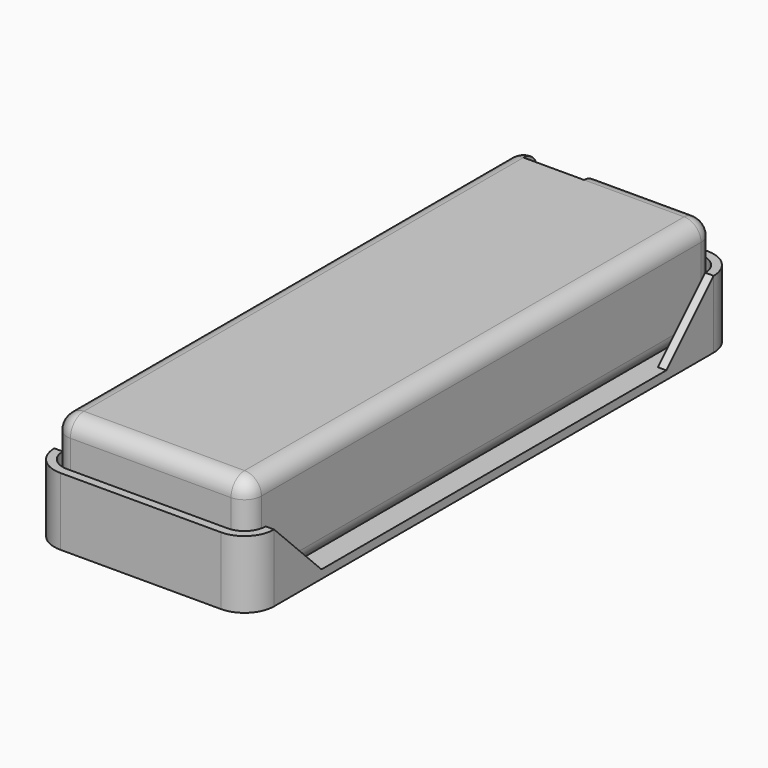
from build123d import *

# Parameters (mm, degrees)
F1_DEPTH  = 24
F2_R      = 4
F3_W      = 14.3697379231
F3_H      = 4.1815820932
F4_DEPTH  = 10
F5_DEPTH  = 14
F6_DEPTH  = 2
F7_DEPTH  = 2
F8_W      = 2
F8_H      = 130
F9_DEPTH  = 14
F10_DEPTH = 14
F11_DEPTH = 14
F12_SIZE  = 13.99999


# Not quite as in the source:
# - a fillet or chamfer is up to 0.001 mm smaller than in the source, because OpenCascade refuses the exact size


with BuildPart() as f1:
    # F0 (on Top) → F1 (new body)
    with BuildSketch(Plane.XY):
        with BuildLine():
            Line((-42, 0), (-4, 0))
            ThreePointArc((-4, 0), (-1.1715728753, 1.1715728753), (0, 4))
            Line((0, 4), (0, 134))
            ThreePointArc((0, 134), (-1.1715728753, 136.8284271247), (-4, 138))
            Line((-4, 138), (-42, 138))
            ThreePointArc((-42, 138), (-44.8284271247, 136.8284271247), (-46, 134))
            Line((-46, 134), (-46, 4))
            ThreePointArc((-46, 4), (-44.8284271247, 1.1715728753), (-42, 0))
        make_face()
    extrude(amount=F1_DEPTH)

    # F2
    f2_edges = [f1.edges().sort_by_distance(p)[0] for p in [
        (-46, 69, 24),
        (-44.828427, 1.171573, 24),
        (-23, 0, 24),
        (-1.171573, 1.171573, 24),
        (0, 69, 24),
        (-1.171573, 136.828427, 24),
        (-23, 138, 24),
        (-44.828427, 136.828427, 24),
        (-46, 69, 0),
        (-44.828427, 1.171573, 0),
        (-23, 0, 0),
        (-1.171573, 1.171573, 0),
        (0, 69, 0),
        (-1.171573, 136.828427, 0),
        (-23, 138, 0),
        (-44.828427, 136.828427, 0),
    ]]
    fillet(f2_edges, radius=F2_R)

    # F3 (on face) → F4 (cut)
    with BuildSketch(Plane.XY.offset(24)):
        with Locations((-34.8151310384, 136.0907910466)):
            Rectangle(F3_W, F3_H)
    extrude(amount=-F4_DEPTH, mode=Mode.SUBTRACT)


with BuildPart() as f5:
    # F0 (on Top) → F5 (new body)
    with BuildSketch(Plane.XY):
        with BuildLine():
            Line((-42, -3), (-4, -3))
            ThreePointArc((-4, -3), (0.9497474683, -0.9497474683), (3, 4))
            Line((3, 4), (3, 134))
            ThreePointArc((3, 134), (0.9497474683, 138.9497474683), (-4, 141))
            Line((-4, 141), (-42, 141))
            ThreePointArc((-42, 141), (-46.9497474683, 138.9497474683), (-49, 134))
            Line((-49, 134), (-49, 4))
            ThreePointArc((-49, 4), (-46.9497474683, -0.9497474683), (-42, -3))
        make_face()
        with BuildLine():
            ThreePointArc((-42, -1), (-45.5355339059, 0.4644660941), (-47, 4))
            Line((-47, 4), (-47, 134))
            ThreePointArc((-47, 134), (-45.5355339059, 137.5355339059), (-42, 139))
            Line((-42, 139), (-4, 139))
            ThreePointArc((-4, 139), (-0.4644660941, 137.5355339059), (1, 134))
            Line((1, 134), (1, 4))
            ThreePointArc((1, 4), (-0.4644660941, 0.4644660941), (-4, -1))
            Line((-4, -1), (-42, -1))
        make_face(mode=Mode.SUBTRACT)
    extrude(amount=F5_DEPTH)



with BuildPart() as f6:
    # F0 (on Top) → F6 (new body)
    with BuildSketch(Plane.XY):
        with BuildLine():
            Line((-42, -3), (-4, -3))
            ThreePointArc((-4, -3), (0.9497474683, -0.9497474683), (3, 4))
            Line((3, 4), (3, 134))
            ThreePointArc((3, 134), (0.9497474683, 138.9497474683), (-4, 141))
            Line((-4, 141), (-42, 141))
            ThreePointArc((-42, 141), (-46.9497474683, 138.9497474683), (-49, 134))
            Line((-49, 134), (-49, 4))
            ThreePointArc((-49, 4), (-46.9497474683, -0.9497474683), (-42, -3))
        make_face()
        with BuildLine():
            ThreePointArc((-42, -1), (-45.5355339059, 0.4644660941), (-47, 4))
            Line((-47, 4), (-47, 134))
            ThreePointArc((-47, 134), (-45.5355339059, 137.5355339059), (-42, 139))
            Line((-42, 139), (-4, 139))
            ThreePointArc((-4, 139), (-0.4644660941, 137.5355339059), (1, 134))
            Line((1, 134), (1, 4))
            ThreePointArc((1, 4), (-0.4644660941, 0.4644660941), (-4, -1))
            Line((-4, -1), (-42, -1))
        make_face(mode=Mode.SUBTRACT)
    extrude(amount=-F6_DEPTH)


with BuildPart() as f6b:
    # F0 (on Top) → F6, piece 2 (new body)
    with BuildSketch(Plane.XY):
        with BuildLine():
            Line((-42, 0), (-4, 0))
            ThreePointArc((-4, 0), (-1.1715728753, 1.1715728753), (0, 4))
            Line((0, 4), (0, 134))
            ThreePointArc((0, 134), (-1.1715728753, 136.8284271247), (-4, 138))
            Line((-4, 138), (-42, 138))
            ThreePointArc((-42, 138), (-44.8284271247, 136.8284271247), (-46, 134))
            Line((-46, 134), (-46, 4))
            ThreePointArc((-46, 4), (-44.8284271247, 1.1715728753), (-42, 0))
        make_face()
    extrude(amount=-F6_DEPTH)


with BuildPart() as f5_1:
    add(f5.part)

    add(f6.part)  # F7 merges F6

    add(f6b.part)  # F7 merges F6b
    # F0 (on Top) → F7 (join)
    with BuildSketch(Plane.XY):
        with BuildLine():
            Line((-47, 134), (-47, 4))
            ThreePointArc((-47, 4), (-45.5355339059, 0.4644660941), (-42, -1))
            Line((-42, -1), (-4, -1))
            ThreePointArc((-4, -1), (-0.4644660941, 0.4644660941), (1, 4))
            Line((1, 4), (1, 134))
            ThreePointArc((1, 134), (-0.4644660941, 137.5355339059), (-4, 139))
            Line((-4, 139), (-42, 139))
            ThreePointArc((-42, 139), (-45.5355339059, 137.5355339059), (-47, 134))
        make_face()
        with BuildLine():
            ThreePointArc((0, 4), (-1.1715728753, 1.1715728753), (-4, 0))
            Line((-4, 0), (-42, 0))
            ThreePointArc((-42, 0), (-44.8284271247, 1.1715728753), (-46, 4))
            Line((-46, 4), (-46, 134))
            ThreePointArc((-46, 134), (-44.8284271247, 136.8284271247), (-42, 138))
            Line((-42, 138), (-4, 138))
            ThreePointArc((-4, 138), (-1.1715728753, 136.8284271247), (0, 134))
            Line((0, 134), (0, 4))
        make_face(mode=Mode.SUBTRACT)
    extrude(amount=-F7_DEPTH)

    # F8 (on face) → F9 (cut)
    with BuildSketch(Plane.XY.offset(14)):
        with Locations((-48, 69)):
            Rectangle(F8_W, F8_H)
        with Locations((2, 69)):
            Rectangle(F8_W, F8_H)
    extrude(amount=-F9_DEPTH, mode=Mode.SUBTRACT)

    # F10 (add): faces of the model
    f10_faces = [f5_1.faces().sort_by_distance(p)[0] for p in [
        (-48, 4, 7),
        (2, 4, 7),
    ]]
    extrude(f10_faces, amount=F10_DEPTH)

    # F11 (add): faces of the model
    f11_faces = [f5_1.faces().sort_by_distance(p)[0] for p in [
        (2, 134, 7),
        (-48, 134, 7),
    ]]
    extrude(f11_faces, amount=F11_DEPTH)

    # F12 (size 14 in the source; OpenCascade refuses exactly that, so slightly less here)
    f12_edges = [f5_1.edges().sort_by_distance(p)[0] for p in [
        (-48, 120, 14),
        (2, 120, 14),
        (2, 18, 14),
        (-48, 18, 14),
    ]]
    chamfer(f12_edges, length=F12_SIZE)


solid = Compound([f1.part, f5_1.part])
